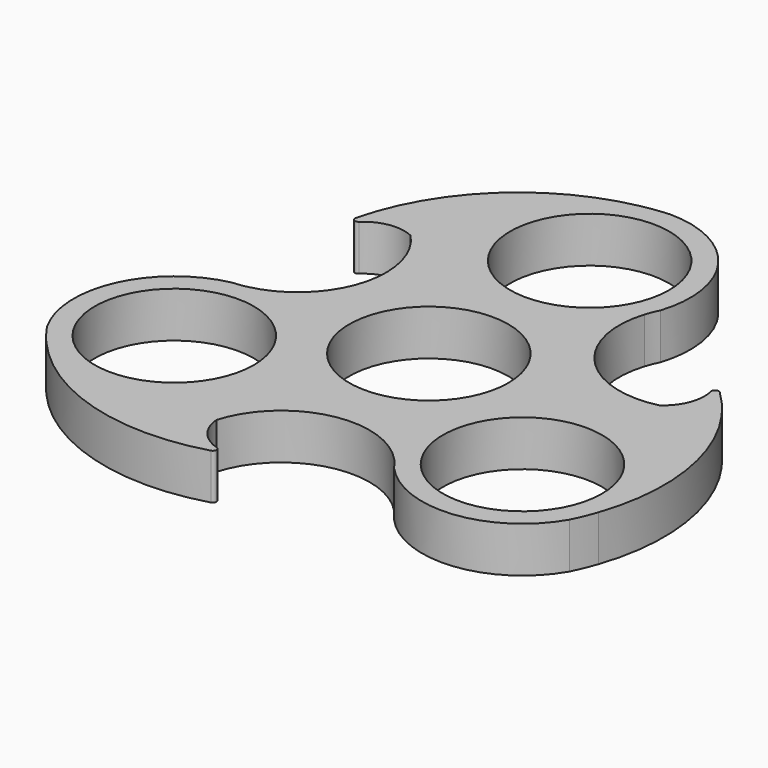
from build123d import *

# Parameters (mm, degrees)
F0_R     = 11.05
F1_DEPTH = 6.35
F2_R     = 0.508


# Not quite as in the source:
# - a feature names something its author has since deleted; it is built from what else it names


with BuildPart() as f1:
    # F0 (on Top) → F1 (new body)
    with BuildSketch(Plane.XY):
        with BuildLine():
            ThreePointArc((27.1429276567, 6.1352837814), (15.2810658667, 9.7013912391), (12.5387063316, 21.7803130331))
            ThreePointArc((12.5387063316, 21.7803130331), (12.8751071514, 22.7165186649), (13.2860771432, 23.6224712919))
            ThreePointArc((13.2860771432, 23.6224712919), (11.3021408603, 36.1511212373), (0, 41.91))
            ThreePointArc((0, 41.91), (-1.8008358417, 41.7320810261), (-3.5869805559, 41.4416469548))
            ThreePointArc((-3.5869805559, 41.4416469548), (-18.8414291839, 33.1449919843), (-26.5736300498, 17.5968166441))
            ThreePointArc((-26.5736300498, 17.5968166441), (-23.32919107, 20.6410473634), (-18.8847754424, 20.4388229931))
            ThreePointArc((-18.8847754424, 20.4388229931), (-16.0421841985, 8.3830956179), (-25.1316575548, -0.0313183028))
            ThreePointArc((-25.1316575548, -0.0313183028), (-26.1106358251, -0.2080894629), (-27.1006988106, -0.3051553233))
            ThreePointArc((-27.1006988106, -0.3051553233), (-36.958859797, -8.2876195165), (-36.2951246726, -20.955))
            ThreePointArc((-36.2951246726, -20.955), (-35.2406244005, -22.4256101), (-34.0960287596, -23.8272397617))
            ThreePointArc((-34.0960287596, -23.8272397617), (-19.2836904747, -32.889652309), (-1.9524752146, -31.811847016))
            ThreePointArc((-1.9524752146, -31.811847016), (-6.2110758425, -30.5241957981), (-8.2581522143, -26.5741067745))
            ThreePointArc((-8.2581522143, -26.5741067745), (0.7611183318, -18.0844868571), (12.5929512232, -21.7489947303))
            ThreePointArc((12.5929512232, -21.7489947303), (13.2355286736, -22.508429202), (13.8146216674, -23.3173159686))
            ThreePointArc((13.8146216674, -23.3173159686), (25.6567189367, -27.8635017208), (36.2951246726, -20.955))
            ThreePointArc((36.2951246726, -20.955), (37.0414602422, -19.3064709261), (37.6830093155, -17.6144071931))
            ThreePointArc((37.6830093155, -17.6144071931), (38.1251196586, -0.2553396753), (28.5261052644, 14.2150303719))
            ThreePointArc((28.5261052644, 14.2150303719), (29.5402669125, 9.8831484346), (27.1429276567, 6.1352837814))
        make_face()
        with Locations((-24.1967497817, -13.97)):
            Circle(F0_R, mode=Mode.SUBTRACT)
        Circle(F0_R, mode=Mode.SUBTRACT)
        with Locations((24.1967497817, -13.97)):
            Circle(F0_R, mode=Mode.SUBTRACT)
        with Locations((0, 27.94)):
            Circle(F0_R, mode=Mode.SUBTRACT)
    extrude(amount=F1_DEPTH)

    # F2
    f2_edges = [f1.edges().sort_by_distance(p)[0] for p in [
        (-1.952475, -31.811847, 3.175),
        (-26.57363, 17.596817, 3.175),
        (28.526105, 14.21503, 3.175),
    ]]
    fillet(f2_edges, radius=F2_R)


solid = f1.part
